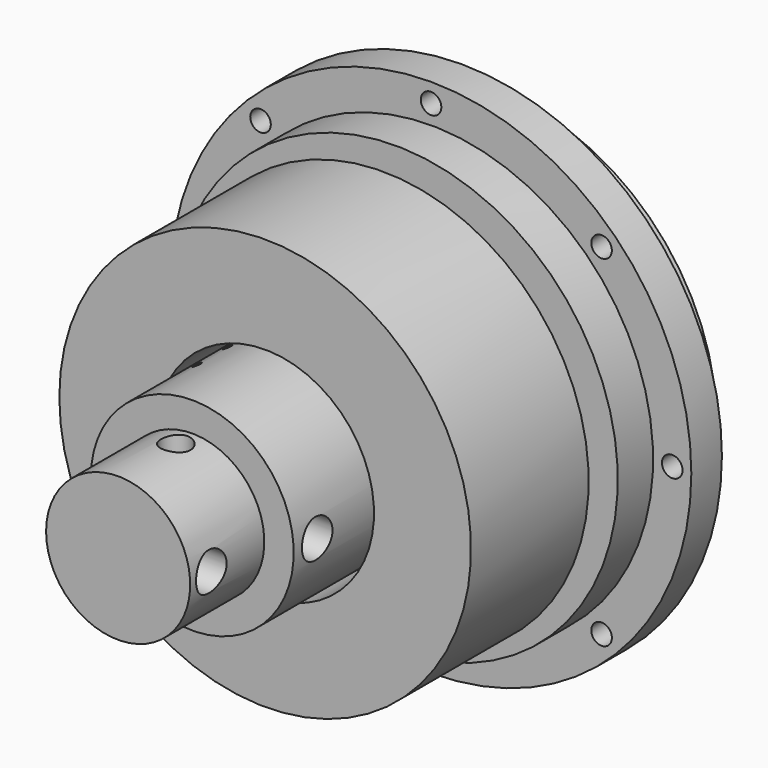
from build123d import *

# Parameters (mm, degrees)
F2_R      = 37
F3_DEPTH  = 5
F4_R      = 55
F4_R_2    = 53
F5_DEPTH  = 3
F6_R      = 50
F6_R_2    = 37
F7_DEPTH  = 5
F8_R      = 62.5
F8_R_2    = 50
F9_DEPTH  = 13
F21_W     = 13
F21_H     = 13
F23_R     = 3.5
F24_DEPTH = 166.001
F25_R     = 3.5
F26_DEPTH = 160.001
F27_R     = 3.5
F28_DEPTH = 146.001
F34_R     = 5
F35_DEPTH = 188.501
F36_R     = 5
F37_REACH = 111.810597333
F38_R     = 6.5
F39_DEPTH = 188.501
F40_DEPTH = 100
F41_R     = 1.5
F42_REACH = 105.1086660909
F43_R     = 5.5
F44_DEPTH = 80.001


with BuildPart() as f1:
    # F0 (on Top) → F1 (revolve)
    with BuildSketch(Plane.XY):
        Polygon((0, -37), (0, 23.5), (-29.5, 23.5), (-29.5, 5), (-32.3867513459, 0), (-50, 0), (-50, -12), (-37, -12), (-37, -30), (-30, -30), (-30, -37), align=None)
    revolve(axis=Axis((0, -6.75, 0), (0, 1, 0)))

    # F23 (on face) → F24 (cut, through all)
    with BuildSketch(Plane(origin=(0, 0, 0), x_dir=(-1, 0, 0), z_dir=(0, 1, 0))):
        with Locations((-43, 0)):
            Circle(F23_R)
        with Locations((-30.405591591, -30.405591591)):
            Circle(F23_R)
        with Locations((0, -43)):
            Circle(F23_R)
        with Locations((30.405591591, -30.405591591)):
            Circle(F23_R)
        with Locations((43, 0)):
            Circle(F23_R)
        with Locations((30.405591591, 30.405591591)):
            Circle(F23_R)
        with Locations((0, 43)):
            Circle(F23_R)
        with Locations((-30.405591591, 30.405591591)):
            Circle(F23_R)
    extrude(amount=-F24_DEPTH, mode=Mode.SUBTRACT)


with BuildPart() as f3:
    # F2 (on face) → F3 (new body)
    with BuildSketch(Plane.XZ.offset(12)):
        with BuildLine():
            ThreePointArc((-55, 0), (0, -55), (55, 0))
            ThreePointArc((55, 0), (0, 55), (-55, 0))
        make_face()
        Circle(F2_R, mode=Mode.SUBTRACT)
    extrude(amount=F3_DEPTH)

    # F4 (on face) → F5 (join)
    with BuildSketch(Plane(origin=(0, -12, 0), x_dir=(-1, 0, 0), z_dir=(0, 1, 0))):
        Circle(F4_R)
        Circle(F4_R_2, mode=Mode.SUBTRACT)
    extrude(amount=F5_DEPTH)

    # F6 (on face) → F7 (join)
    with BuildSketch(Plane.XZ.offset(17)):
        Circle(F6_R)
        Circle(F6_R_2, mode=Mode.SUBTRACT)
    extrude(amount=F7_DEPTH)


with BuildPart() as f9:
    # F8 (on face) → F9 (new body)
    with BuildSketch(Plane.XZ.offset(17)):
        Circle(F8_R)
        Circle(F8_R_2, mode=Mode.SUBTRACT)
    extrude(amount=F9_DEPTH)


with BuildPart() as f10_1:
    # F10: copy of F9
    add(f9.part.moved(Location((0, -13, 0))))


with BuildPart() as f12:
    # F11 (on Top) → F12 (revolve)
    with BuildSketch(Plane.XY):
        Polygon((-62.5, -17), (-57.5, -17), (-57.5, -8.8), (-52.8, -8.8), (-52.8, -11.8), (-50.2, -11.8), (-50.2, -6), (-75.5, -6), (-75.5, -17), (-75.5, -20), (-62.5, -20), align=None)
    revolve(axis=Axis((0, -7.0216925815, 0), (0, 1, 0)))

    # F25 (on face) → F26 (cut, through all)
    with BuildSketch(Plane(origin=(0, -6, 0), x_dir=(-1, 0, 0), z_dir=(0, 1, 0))):
        with Locations((0, 68.5)):
            Circle(F25_R)
        with Locations((-48.4368145113, 48.4368145113)):
            Circle(F25_R)
        with Locations((-68.5, 0)):
            Circle(F25_R)
        with Locations((-48.4368145113, -48.4368145113)):
            Circle(F25_R)
        with Locations((0, -68.5)):
            Circle(F25_R)
        with Locations((48.4368145113, -48.4368145113)):
            Circle(F25_R)
        with Locations((68.5, 0)):
            Circle(F25_R)
        with Locations((48.4368145113, 48.4368145113)):
            Circle(F25_R)
    extrude(amount=-F26_DEPTH, mode=Mode.SUBTRACT)


with BuildPart() as f14:
    # F13 (on Top) → F14 (revolve)
    with BuildSketch(Plane.XY):
        Polygon((-9.5, -48), (-9.5, -38), (-37, -38), (-37, -22), (-50, -22), (-50, -43), (-55, -43), (-57, -45), (-57, -51), (-54, -51), (-54, -48), align=None)
    revolve(axis=Axis((0, -43, 0), (0, 1, 0)))


with BuildPart() as f16:
    # F15 (on Top) → F16 (revolve)
    with BuildSketch(Plane.XY):
        Polygon((-54, -56.5), (-3, -56.5), (-3, -38.3), (-9.5, -38.3), (-9.5, -40.5358983849), (-7.5, -48), (-7.5, -51), (-30.5, -51), (-32.5, -51), (-32.5, -49.5), (-32.5, -48), (-54, -48), align=None)
        with BuildLine():
            add(Edge.make_bspline(
                [(-32.5, -49.5), (-32.5, -51), (-30.5, -51)],
                knots=[0, 0, 0, 1.5707963268, 1.5707963268, 1.5707963268], degree=2, weights=[1, 0.7071067812, 1]))
            Line((-32.5, -49.5), (-32.5, -51))
            Line((-32.5, -51), (-30.5, -51))
        make_face()
        with BuildLine():
            add(Edge.make_bspline(
                [(-30.5, -51), (-25.6715728753, -51), (-29.0857864376, -48.4393398282), (-32.5, -45.8786796564), (-32.5, -49.5)],
                knots=[1.5707963268, 1.5707963268, 1.5707963268, 3.926990817, 3.926990817, 6.2831853072, 6.2831853072, 6.2831853072], degree=2, weights=[1, 0.3826834324, 1, 0.3826834324, 1]))
            add(Edge.make_bspline(
                [(-32.5, -49.5), (-32.5, -51), (-30.5, -51)],
                knots=[0, 0, 0, 1.5707963268, 1.5707963268, 1.5707963268], degree=2, weights=[1, 0.7071067812, 1]))
        make_face()
    revolve(axis=Axis((0, -52.25, 0), (0, 1, 0)))

    # F43 (on face) → F44 (cut, through all)
    with BuildSketch(Plane.XZ.offset(56.5)):
        with Locations((-45.25, 0)):
            Circle(F43_R)
        with Locations((0, -45.25)):
            Circle(F43_R)
        with Locations((45.25, 0)):
            Circle(F43_R)
        with Locations((0, 45.25)):
            Circle(F43_R)
    extrude(amount=-F44_DEPTH, mode=Mode.SUBTRACT)


with BuildPart() as f18:
    # F17 (on Top) → F18 (revolve)
    with BuildSketch(Plane.XY):
        Polygon((0, -91.5), (0, -66.5), (-3, -66.5), (-3, -56.5), (-34.5, -56.5), (-34.5, -91), (-34, -91.5), align=None)
        Polygon((0, -134.5), (0, -91.5), (-34, -91.5), (-34.5, -92), (-34.5, -134.5), (-24.5, -134.5), (-24.5, -166), (0, -166), align=None)
    revolve(axis=Axis((0, -100.5, 0), (0, 1, 0)))

    # F34 (on line) → F35 (cut, through all)
    with BuildSketch(Plane.XY.offset(-100)):
        with Locations((0, -141.5)):
            Circle(F34_R)
    extrude(amount=F35_DEPTH, mode=Mode.SUBTRACT)

    f37_end = Plane.XY
    # F36 (on line) → F37 (cut, up to a plane its end follows)
    with BuildSketch(Plane(origin=(42.2618261741, 0, -90.6307787037), x_dir=(0.906307787, 0, 0.4226182617), z_dir=(-0.4226182617, 0, 0.906307787))):
        with Locations((0, -108.5)):
            Circle(F36_R)
    f37_long = extrude(amount=F37_REACH, mode=Mode.PRIVATE)
    add(split(f37_long, bisect_by=f37_end, keep=Keep.BOTTOM, mode=Mode.PRIVATE), mode=Mode.SUBTRACT)

    # F38 (on line) → F39 (cut, through all)
    with BuildSketch(Plane.YZ.offset(100)):
        with Locations((-124.5, 0)):
            Circle(F38_R)
    extrude(amount=-F39_DEPTH, mode=Mode.SUBTRACT)

    # F38 (on line) → F40 (cut, through all)
    with BuildSketch(Plane.YZ.offset(100)):
        with Locations((-157, 0)):
            Circle(F38_R)
    extrude(amount=-F40_DEPTH, mode=Mode.SUBTRACT)

    f42_end = Plane.XY
    # F41 (on line) → F42 (cut, up to a plane its end follows)
    with BuildSketch(Plane(origin=(-50, 0, 86.6025403784), x_dir=(0.8660254038, 0, 0.5), z_dir=(-0.5, 0, 0.8660254038))):
        with Locations((0, -98)):
            Circle(F41_R)
        with Locations((0, -111)):
            Circle(F41_R)
    f42_long = extrude(amount=-F42_REACH, mode=Mode.PRIVATE)
    add(split(f42_long, bisect_by=f42_end, keep=Keep.TOP, mode=Mode.PRIVATE), mode=Mode.SUBTRACT)


with BuildPart() as f20:
    # F19 (on Top) → F20 (revolve)
    with BuildSketch(Plane.XY):
        Polygon((-37, -103.5), (-37, -56.5), (-54, -56.5), (-54, -53.5), (-70, -53.5), (-70, -103.5), align=None)
    revolve(axis=Axis((0, -80, 0), (0, -1, 0)))


with BuildPart() as f22:
    # F21 (on Top) → F22 (revolve)
    with BuildSketch(Plane.XY):
        Polygon((-58.5, -48), (-58.5, -43), (-62.5, -43), (-62.5, -20), (-75.5, -20), (-75.5, -33), (-75.5, -48), align=None)
        with Locations((-82, -26.5)):
            Rectangle(F21_W, F21_H)
    revolve(axis=Axis((0, -28.4441411495, 0), (0, -1, 0)))

    # F27 (on face) → F28 (cut, through all)
    with BuildSketch(Plane(origin=(0, -20, 0), x_dir=(-1, 0, 0), z_dir=(0, 1, 0))):
        with Locations((0, 82)):
            Circle(F27_R)
        with Locations((-57.9827560573, 57.9827560573)):
            Circle(F27_R)
        with Locations((-82, 0)):
            Circle(F27_R)
        with Locations((-57.9827560573, -57.9827560573)):
            Circle(F27_R)
        with Locations((0, -82)):
            Circle(F27_R)
        with Locations((57.9827560573, -57.9827560573)):
            Circle(F27_R)
        with Locations((82, 0)):
            Circle(F27_R)
        with Locations((57.9827560573, 57.9827560573)):
            Circle(F27_R)
    extrude(amount=-F28_DEPTH, mode=Mode.SUBTRACT)


solid = Compound([f1.part, f3.part, f9.part, f10_1.part, f12.part, f14.part, f16.part, f18.part, f20.part, f22.part])
